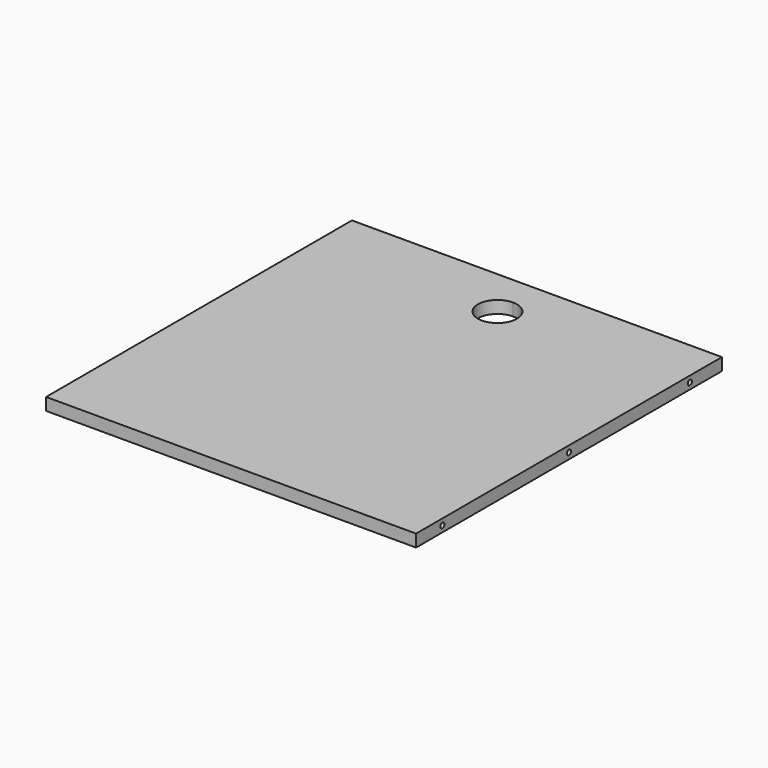
from build123d import *

# Parameters (mm, degrees)
F1_DEPTH  = 19.05
F3_D      = 15.0114
F3_DEPTH  = 14.224
F3_TIP    = 4.5098795482
F5_D      = 8.001
F5_DEPTH  = 25.4
F5_TIP    = 2.4037429064
F7_D      = 8.001
F7_DEPTH  = 25.4
F7_TIP    = 2.4037429064
F9_D      = 8.001
F9_DEPTH  = 14.224
F9_TIP    = 2.4037429064
F11_D     = 15.0114
F11_DEPTH = 14.224
F11_TIP   = 4.5098795482


# Not quite as in the source:
# - a feature names something its author has since deleted; it is built from what else it names


with BuildPart() as f1:
    # F0 (on Top) → F1 (new body)
    with BuildSketch(Plane.XY):
        Polygon((285.75, -295.275), (285.75, 295.275), (0, 295.275), (-285.75, 295.275), (-285.75, -295.275), align=None)
        with BuildLine():
            ThreePointArc((30.1625, 219.075), (-21.3281082875, 197.7468917125), (0, 249.2375))
            ThreePointArc((0, 249.2375), (21.3281082875, 240.4031082875), (30.1625, 219.075))
        make_face(mode=Mode.SUBTRACT)
    extrude(amount=F1_DEPTH)

    # F3
    with Locations(Plane(origin=(0, 0, 0), x_dir=(1, 0, 0), z_dir=(0, 0, -1))):
        with Locations((-261.874, 244.475), (261.874, 244.475), (-261.874, 0), (261.874, 0), (261.874, -244.475), (-261.874, -244.475)):
            Hole(F3_D / 2, depth=F3_DEPTH)
            with Locations((0, 0, -(F3_DEPTH + F3_TIP / 2))):  # 118° drill point
                Cone(0, F3_D / 2, F3_TIP, mode=Mode.SUBTRACT)

    # F5
    with Locations(Plane.YZ.offset(285.75)):
        with Locations((-244.475, 9.525), (0, 9.525), (233.3625, 9.525)):
            Hole(F5_D / 2, depth=F5_DEPTH)
            with Locations((0, 0, -(F5_DEPTH + F5_TIP / 2))):  # 118° drill point
                Cone(0, F5_D / 2, F5_TIP, mode=Mode.SUBTRACT)

    # F7
    with Locations(Plane(origin=(-285.75, 0, 0), x_dir=(0, -1, 0), z_dir=(-1, 0, 0))):
        with Locations((0, 9.525), (244.475, 9.525), (-244.475, 9.525)):
            Hole(F7_D / 2, depth=F7_DEPTH)
            with Locations((0, 0, -(F7_DEPTH + F7_TIP / 2))):  # 118° drill point
                Cone(0, F7_D / 2, F7_TIP, mode=Mode.SUBTRACT)

    # F9
    with Locations(Plane(origin=(0, 0, 0), x_dir=(1, 0, 0), z_dir=(0, 0, -1))):
        with Locations((-234.95, 279.4), (0, 279.4), (234.95, 279.4)):
            Hole(F9_D / 2, depth=F9_DEPTH)
            with Locations((0, 0, -(F9_DEPTH + F9_TIP / 2))):  # 118° drill point
                Cone(0, F9_D / 2, F9_TIP, mode=Mode.SUBTRACT)

    # F11
    with Locations(Plane(origin=(0, 0, 0), x_dir=(1, 0, 0), z_dir=(0, 0, -1))):
        with Locations((-234.95, -271.399), (234.95, -271.399)):
            Hole(F11_D / 2, depth=F11_DEPTH)
            with Locations((0, 0, -(F11_DEPTH + F11_TIP / 2))):  # 118° drill point
                Cone(0, F11_D / 2, F11_TIP, mode=Mode.SUBTRACT)


solid = f1.part
